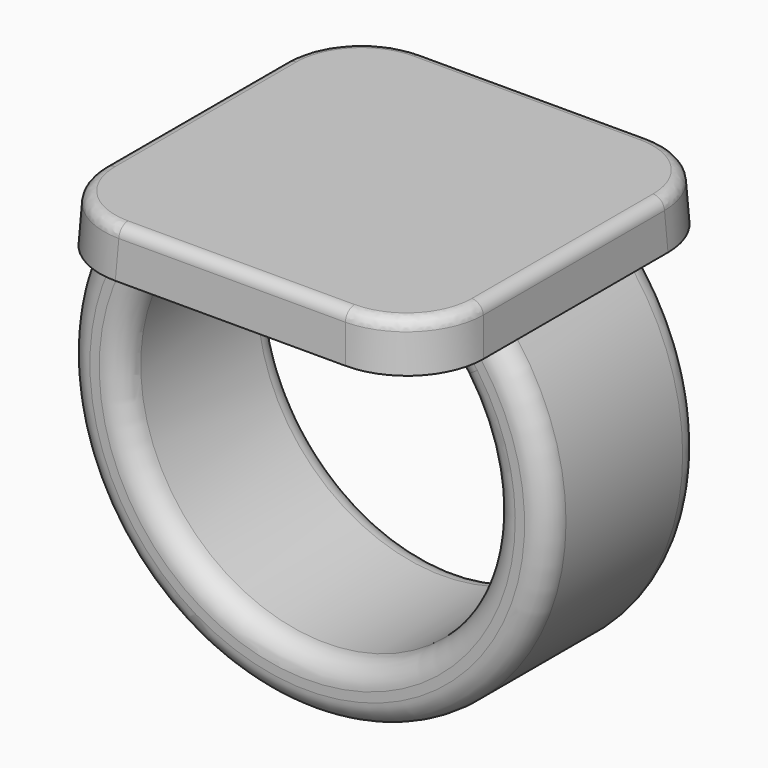
from build123d import *

# Parameters (mm, degrees)
F0_W          = 25.4
F0_H          = 25.4
F1_DEPTH      = 3.175
F1_TAPER      = 3
F3_W          = 5.08
F3_H          = 12.7
F6_DEPTH      = 6.35
F6_DEPTH_BACK = 6.35
F7_R          = 5.08
F8_R          = 1.524
F9_R          = 0.762


with BuildPart() as f1:
    # F0 (on Top) → F1 (new body)
    with BuildSketch(Plane.XY):
        Rectangle(F0_W, F0_H)
    extrude(amount=F1_DEPTH, taper=F1_TAPER)

    # F4: sweep along a path in F2
    with BuildLine(Plane.XZ) as f4_path:
        ThreePointArc((-10.16, 0), (0, -23.5582897328), (10.16, 0))
    # F3 (on face) → F4 (sweep)
    with BuildSketch(Plane(origin=(0, 0, 0), x_dir=(1, 0, 0), z_dir=(0, 0, -1))):
        with Locations((-10.16, 0)):
            Rectangle(F3_W, F3_H)
    sweep(path=f4_path.line)

    # F5 (on Front) → F6 (join, two sides)
    with BuildSketch(Plane.XZ) as f6_sk:
        with BuildLine():
            Line((10.0130578512, -2.535746045), (10.16, 0))
            Line((10.16, 0), (7.62, 0))
            ThreePointArc((7.62, 0), (8.9072265211, -1.1822790439), (10.0130578512, -2.535746045))
        make_face()
    extrude(amount=F6_DEPTH)
    extrude(f6_sk.sketch, amount=-F6_DEPTH_BACK)

    # F7
    f7_edges = [f1.edges().sort_by_distance(p)[0] for p in [
        (12.616803, -12.616803, 1.5875),
        (12.616803, 12.616803, 1.5875),
        (-12.616803, 12.616803, 1.5875),
        (-12.616803, -12.616803, 1.5875),
    ]]
    fillet(f7_edges, radius=F7_R)

    # F8
    f8_edges = [f1.edges().sort_by_distance(p)[0] for p in [
        (-1.743325, 6.35, -21.711017),
        (-1.743325, -6.35, -21.711017),
        (8.907227, -6.35, -1.182279),
        (0, -6.35, -25.501344),
        (0, 6.35, -25.501344),
        (8.907227, 6.35, -1.182279),
    ]]
    fillet(f8_edges, radius=F8_R)

    # F9
    f9_edges = [f1.edges().sort_by_distance(p)[0] for p in [
        (12.533605, 0, 3.175),
        (11.048589, -11.048589, 3.175),
        (11.048589, 11.048589, 3.175),
        (0, -12.533605, 3.175),
        (0, 12.533605, 3.175),
        (-11.048589, -11.048589, 3.175),
        (-11.048589, 11.048589, 3.175),
        (-12.533605, 0, 3.175),
    ]]
    fillet(f9_edges, radius=F9_R)


solid = f1.part
